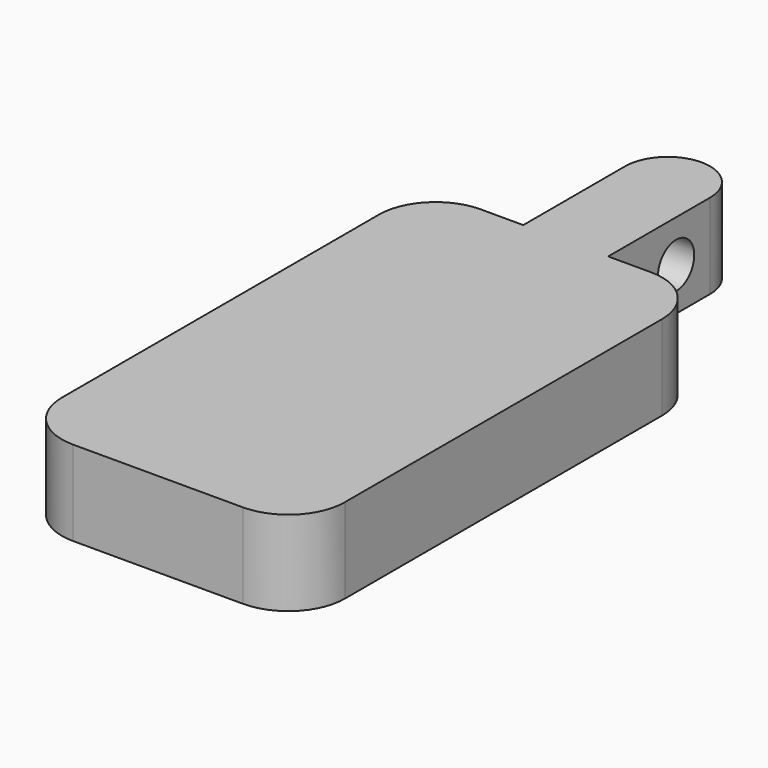
from build123d import *

# Parameters (mm, degrees)
F1_DEPTH = 15
F2_R     = 7.49999
F3_R     = 10
F4_R     = 4
F5_DEPTH = 15


# Not quite as in the source:
# - a fillet or chamfer is up to 0.001 mm smaller than in the source, because OpenCascade refuses the exact size


with BuildPart() as f1:
    # F0 (on Top) → F1 (new body)
    with BuildSketch(Plane.XY):
        Polygon((0, 90), (0, 0), (50, 0), (50, 90), (32.5, 90), (32.5, 120), (17.5, 120), (17.5, 90), align=None)
    extrude(amount=F1_DEPTH)

    # F2 (radius 7.5 in the source; OpenCascade refuses exactly that, so slightly less here)
    f2_edges = [f1.edges().sort_by_distance(p)[0] for p in [
        (17.5, 120, 7.5),
        (32.5, 120, 7.5),
    ]]
    fillet(f2_edges, radius=F2_R)

    # F3
    f3_edges = [f1.edges().sort_by_distance(p)[0] for p in [
        (0, 90, 7.5),
        (50, 90, 7.5),
        (50, 0, 7.5),
        (0, 0, 7.5),
    ]]
    fillet(f3_edges, radius=F3_R)

    # F4 (on face) → F5 (cut)
    with BuildSketch(Plane.YZ.offset(32.5)):
        with Locations((105, 7.5)):
            Circle(F4_R)
    extrude(amount=-F5_DEPTH, mode=Mode.SUBTRACT)


solid = f1.part
